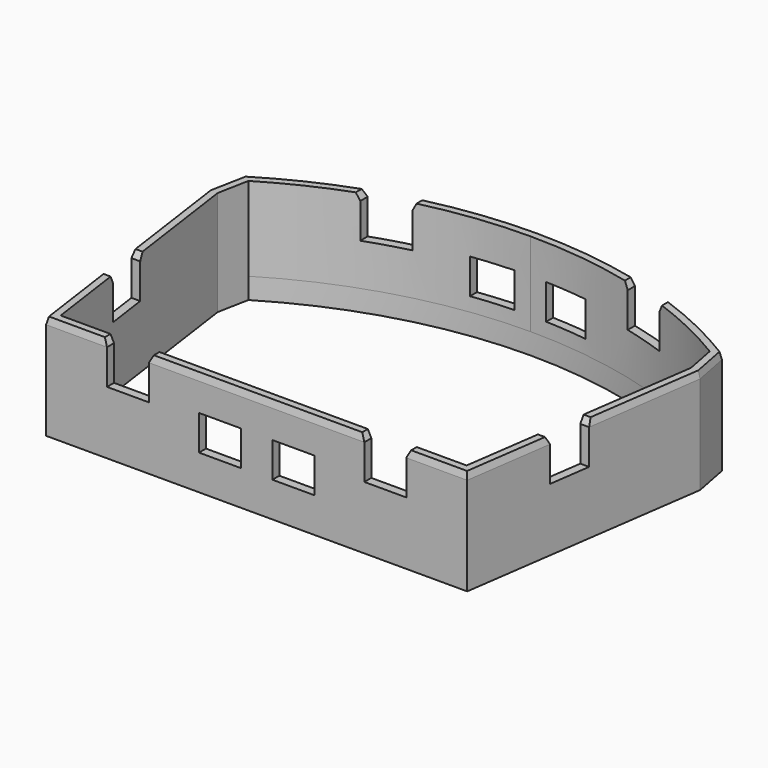
from build123d import *

# Parameters (mm, degrees)
F1_DEPTH     = 12
F2_T1_DEPTH  = 40.9442549995
F2_T3_DEPTH  = 65.4442549995
F2_T5_DEPTH  = 40.9442549995
F2_T7_DEPTH  = 10.4442549995
F2_T9_DEPTH  = 10.4442549995
F2_T12_ANGLE = 68.042658845
F3_W         = 6
F3_H         = 5
F4_DEPTH     = 50.251
F8_DEPTH     = 70.251
F10_DEPTH    = 3


# Not quite as in the source:
# - a fillet or chamfer that OpenCascade refuses, or shapes differently, is made with other operations: its cross-section is extruded or revolved along the edge and cut away or added


with BuildPart() as f1:
    # F0 (on Top) → F1 (new body)
    with BuildSketch(Plane.XY):
        with BuildLine():
            Line((-35.125, 35.3986228546), (-30.125, 0))
            Line((-30.125, 0), (0, 0))
            Line((0, 0), (0, 1.25))
            Line((0, 1.25), (-29.0391526732, 1.25))
            Line((-29.0391526732, 1.25), (-33.8579983297, 35.3660999978))
            Line((-33.8579983297, 35.3660999978), (-33.0027387168, 39.7740071493))
            ThreePointArc((-33.0027387168, 39.7740071493), (-17.1340283274, 46.6501181236), (0, 49))
            Line((0, 49), (0, 50.25))
            ThreePointArc((0, 50.25), (-17.738073715, 47.7785625378), (-34.125, 40.5525048866))
            Line((-34.125, 40.5525048866), (-35.125, 35.3986228546))
        make_face()
        with BuildLine():
            Line((0, 1.25), (0, 0))
            Line((0, 0), (30.125, 0))
            Line((30.125, 0), (35.125, 35.3986228546))
            Line((35.125, 35.3986228546), (34.125, 40.5525048866))
            ThreePointArc((34.125, 40.5525048866), (17.738073715, 47.7785625378), (0, 50.25))
            Line((0, 50.25), (0, 49))
            ThreePointArc((0, 49), (17.1340283274, 46.6501181236), (33.0027387168, 39.7740071493))
            Line((33.0027387168, 39.7740071493), (33.8579983297, 35.3660999978))
            Line((33.8579983297, 35.3660999978), (29.0391526732, 1.25))
            Line((29.0391526732, 1.25), (0, 1.25))
        make_face()
    extrude(amount=F1_DEPTH)

    # F2: chamfer of 0.25 x 1 on 6 edges, made by hand

    # F2_s2 → F2_t1 (cut)
    with BuildSketch(Plane(origin=(-5.9525054843, 42.142099336, 0), x_dir=(0, 0, 1), z_dir=(0.1398601399, -0.9901712687, 0))):
        Polygon((11, 29.8289094684), (12, 29.5789094684), (12, 29.8289094684), align=None)
    extrude(amount=F2_T1_DEPTH, mode=Mode.SUBTRACT)

    # F2_s4 → F2_t3 (cut)
    with BuildSketch(Plane.YZ.offset(-32.7221274998)):
        Polygon((0, 11), (0.25, 12), (0, 12), align=None)
    extrude(amount=F2_T3_DEPTH, mode=Mode.SUBTRACT)

    # F2_s6 → F2_t5 (cut)
    with BuildSketch(Plane(origin=(0.2260362536, 1.6002744188, 0), x_dir=(0, 0, 1), z_dir=(0.1398601399, 0.9901712687, 0))):
        Polygon((11, 29.8289094684), (12, 29.5789094684), (12, 29.8289094684), align=None)
    extrude(amount=F2_T5_DEPTH, mode=Mode.SUBTRACT)

    # F2_s8 → F2_t7 (cut)
    with BuildSketch(Plane(origin=(-4.8500827906, 24.9967545481, 0), x_dir=(0, 0, 1), z_dir=(-0.1904761905, 0.9816918156, 0))):
        Polygon((11, 41.2245198532), (12, 40.9745198532), (12, 41.2245198532), align=None)
    extrude(amount=F2_T7_DEPTH, mode=Mode.SUBTRACT)

    # F2_s10 → F2_t9 (cut)
    with BuildSketch(Plane(origin=(6.8394646952, 35.2497942014, 0), x_dir=(0, 0, 1), z_dir=(-0.1904761905, -0.9816918156, 0))):
        Polygon((11, 41.2245198532), (12, 40.9745198532), (12, 41.2245198532), align=None)
    extrude(amount=F2_T9_DEPTH, mode=Mode.SUBTRACT)

    # F2_s11 → F2_t12 (revolve, cut)
    with BuildSketch(Plane(origin=(6.7894109874, -4.5831938529, 0), x_dir=(0, 0, 1), z_dir=(0.8288293451, -0.5595014894, 0))):
        Polygon((11, -52.7560806603), (12, -52.5060806603), (12, -52.7560806603), align=None)
    revolve(axis=Axis((0, -14.6408311763, 12), (0, 0, 1)), revolution_arc=F2_T12_ANGLE, mode=Mode.SUBTRACT)

    # F3 (on face) → F4 (cut, through all)
    with BuildSketch(Plane.XZ):
        with Locations((-18.4078305346, 8.5)):
            Rectangle(F3_W, F3_H)
        Polygon((-21.9078305346, 12), (-21.4078305346, 11), (-15.4078305346, 11), (-14.9078305346, 12), align=None)
        with Locations((18.4078305346, 8.5)):
            Rectangle(F3_W, F3_H)
        Polygon((14.9078305346, 12), (15.4078305346, 11), (21.4078305346, 11), (21.9078305346, 12), align=None)
        with Locations((-5.25, 4.5)):
            Rectangle(F3_W, F3_H)
        with Locations((5.25, 4.5)):
            Rectangle(F3_W, F3_H)
    extrude(amount=-F4_DEPTH, mode=Mode.SUBTRACT)

    # F7 (on face) → F8 (cut, through all)
    with BuildSketch(Plane(origin=(-35.125, 0, 0), x_dir=(0, -1, 0), z_dir=(-1, 0, 0))):
        Polygon((-19.0282890696, 12), (-18.5332034352, 11), (-18.5332034352, 6), (-12.5921758233, 6), (-12.5921758233, 11), (-12.0970901889, 12), align=None)
    extrude(amount=-F8_DEPTH, mode=Mode.SUBTRACT)

    # F9 (on face) + F0 (on Top) → F10 (join)
    with BuildSketch(Plane(origin=(0, 0, 0), x_dir=(1, 0, 0), z_dir=(0, 0, -1))):
        with BuildLine():
            Line((30.125, 0), (-30.125, 0))
            Line((-30.125, 0), (-35.125, -35.3986228546))
            Line((-35.125, -35.3986228546), (-34.125, -40.5525048866))
            ThreePointArc((-34.125, -40.5525048866), (0, -50.25), (34.125, -40.5525048866))
            Line((34.125, -40.5525048866), (35.125, -35.3986228546))
            Line((35.125, -35.3986228546), (30.125, 0))
        make_face()
        with BuildLine():
            Line((-33.8579983297, -35.3660999978), (-29.0391526732, -1.25))
            Line((-29.0391526732, -1.25), (29.0391526732, -1.25))
            Line((29.0391526732, -1.25), (33.8579983297, -35.3660999978))
            Line((33.8579983297, -35.3660999978), (33.0027387168, -39.7740071493))
            ThreePointArc((33.0027387168, -39.7740071493), (0, -49), (-33.0027387168, -39.7740071493))
            Line((-33.0027387168, -39.7740071493), (-33.8579983297, -35.3660999978))
        make_face(mode=Mode.SUBTRACT)
    with BuildSketch(Plane.XY):
        with BuildLine():
            Line((-35.125, 35.3986228546), (-30.125, 0))
            Line((-30.125, 0), (0, 0))
            Line((0, 0), (0, 1.25))
            Line((0, 1.25), (-29.0391526732, 1.25))
            Line((-29.0391526732, 1.25), (-33.8579983297, 35.3660999978))
            Line((-33.8579983297, 35.3660999978), (-33.0027387168, 39.7740071493))
            ThreePointArc((-33.0027387168, 39.7740071493), (-17.1340283274, 46.6501181236), (0, 49))
            Line((0, 49), (0, 50.25))
            ThreePointArc((0, 50.25), (-17.738073715, 47.7785625378), (-34.125, 40.5525048866))
            Line((-34.125, 40.5525048866), (-35.125, 35.3986228546))
        make_face()
        with BuildLine():
            Line((0, 1.25), (0, 0))
            Line((0, 0), (30.125, 0))
            Line((30.125, 0), (35.125, 35.3986228546))
            Line((35.125, 35.3986228546), (34.125, 40.5525048866))
            ThreePointArc((34.125, 40.5525048866), (17.738073715, 47.7785625378), (0, 50.25))
            Line((0, 50.25), (0, 49))
            ThreePointArc((0, 49), (17.1340283274, 46.6501181236), (33.0027387168, 39.7740071493))
            Line((33.0027387168, 39.7740071493), (33.8579983297, 35.3660999978))
            Line((33.8579983297, 35.3660999978), (29.0391526732, 1.25))
            Line((29.0391526732, 1.25), (0, 1.25))
        make_face()
    extrude(amount=F10_DEPTH, dir=(0, 0, -1))


solid = f1.part
